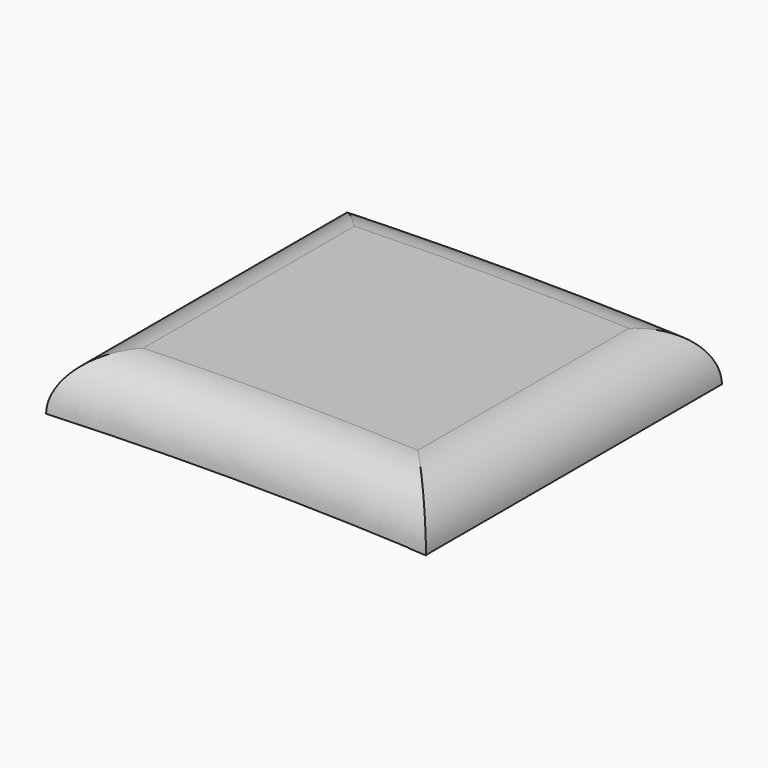
from build123d import *

# Parameters (mm, degrees)
F0_R        = 316.25
F0_R_2      = 281.25
F1_DEPTH    = 10
F3_DEPTH    = 5
F4_W        = 212.0740879327
F4_H        = 34.9558026777
F4_W_2      = 196.2447150651
F4_H_2      = 35.0580604298
F5_DEPTH    = 84
F6_W        = 1.3297378083
F6_H        = 10.0317904726
F7_DEPTH    = 42
F8_T1_DEPTH = 60.0580604298
F8_T3_DEPTH = 60.0708356762
F8_T6_ANGLE = 12.4528096898
F8_T8_ANGLE = 11.0736814867


# Not quite as in the source:
# - a fillet or chamfer that OpenCascade refuses, or shapes differently, is made with other operations: its cross-section is extruded or revolved along the edge and cut away or added


with BuildPart() as f1:
    # F0 (on Top) → F1 (new body)
    with BuildSketch(Plane.XY):
        Circle(F0_R)
        Circle(F0_R_2, mode=Mode.SUBTRACT)
    extrude(amount=F1_DEPTH)

    # F2 (on face) → F3 (join)
    with BuildSketch(Plane.XY.offset(10)):
        with BuildLine():
            ThreePointArc((18.9455430955, 315.6820059757), (0.8957518585, 316.2487314261), (-17.1569601592, 315.7842637278))
            Line((-17.1569601592, 315.7842637278), (-17.1569601592, 280.726203298))
            ThreePointArc((-17.1569601592, 280.726203298), (0.8961391508, 281.2485723246), (18.9455430955, 280.6111702994))
            Line((18.9455430955, 280.6111702994), (18.9455430955, 315.6820059757))
        make_face()
    extrude(amount=F3_DEPTH)

    # F4 (on face) → F5 (cut)
    with BuildSketch(Plane.XY.offset(10)):
        Polygon((417.2187745571, -329.5601010323), (417.2187745571, 280.726203298), (231.0196310282, 280.726203298), (18.9455430955, 280.726203298), (-17.1569601592, 280.726203298), (-213.4016752243, 280.726203298), (-349.9614596367, 280.726203298), (-349.9614596367, -329.5601010323), align=None)
        with Locations((124.9825870618, 298.2041046368)):
            Rectangle(F4_W, F4_H)
        with Locations((-115.2793176918, 298.2552335129)):
            Rectangle(F4_W_2, F4_H_2)
    extrude(amount=-F5_DEPTH, mode=Mode.SUBTRACT)

    # F6 (on face) → F7 (cut)
    with BuildSketch(Plane.YZ.offset(18.9455430955)):
        Polygon((280.726203298, 10), (280.726203298, 0), (315.6820059757, 0), (315.6820059757, 10.0317904726), (280.726203298, 10.0317904726), align=None)
        with Locations((316.3468748798, 5.0158952363)):
            Rectangle(F6_W, F6_H)
    extrude(amount=-F7_DEPTH, mode=Mode.SUBTRACT)

    # F8: fillet of radius 5 on 4 edges, made by hand

    # F8_s2 → F8_t1 (cut)
    with BuildSketch(Plane.XZ.offset(-328.2842637278)):
        with BuildLine():
            ThreePointArc((-17.1569601592, 10), (-15.6924940651, 13.5355339059), (-12.1569601592, 15))
            Line((-12.1569601592, 15), (-17.1569601592, 15))
            Line((-17.1569601592, 15), (-17.1569601592, 10))
        make_face()
    extrude(amount=F8_T1_DEPTH, mode=Mode.SUBTRACT)

    # F8_s4 → F8_t3 (cut)
    with BuildSketch(Plane.XZ.offset(-328.1820059757)):
        with BuildLine():
            ThreePointArc((13.9455430955, 15), (17.4810770014, 13.5355339059), (18.9455430955, 10))
            Line((18.9455430955, 10), (18.9455430955, 15))
            Line((18.9455430955, 15), (13.9455430955, 15))
        make_face()
    extrude(amount=F8_T3_DEPTH, mode=Mode.SUBTRACT)

    # F8_s5 → F8_t6 (revolve, cut)
    with BuildSketch(Plane(origin=(0, 0, 0), x_dir=(0, 0, 1), z_dir=(-0.9944416157, -0.1052894726, 0))):
        with BuildLine():
            ThreePointArc((15, 286.25), (13.5355339059, 282.7144660941), (10, 281.25))
            Line((10, 281.25), (15, 281.25))
            Line((15, 281.25), (15, 286.25))
        make_face()
    revolve(axis=Axis((0, 0, 15), (0, 0, -1)), revolution_arc=F8_T6_ANGLE, mode=Mode.SUBTRACT)

    # F8_s7 → F8_t8 (revolve, cut)
    with BuildSketch(Plane(origin=(0, 0, 0), x_dir=(0, 0, 1), z_dir=(0.995057084, -0.0993045796, 0))):
        with BuildLine():
            ThreePointArc((10, -316.25), (13.5355339059, -314.7855339059), (15, -311.25))
            Line((15, -311.25), (15, -316.25))
            Line((15, -316.25), (10, -316.25))
        make_face()
    revolve(axis=Axis((0, 0, 15), (0, 0, 1)), revolution_arc=F8_T8_ANGLE, mode=Mode.SUBTRACT)


solid = f1.part
